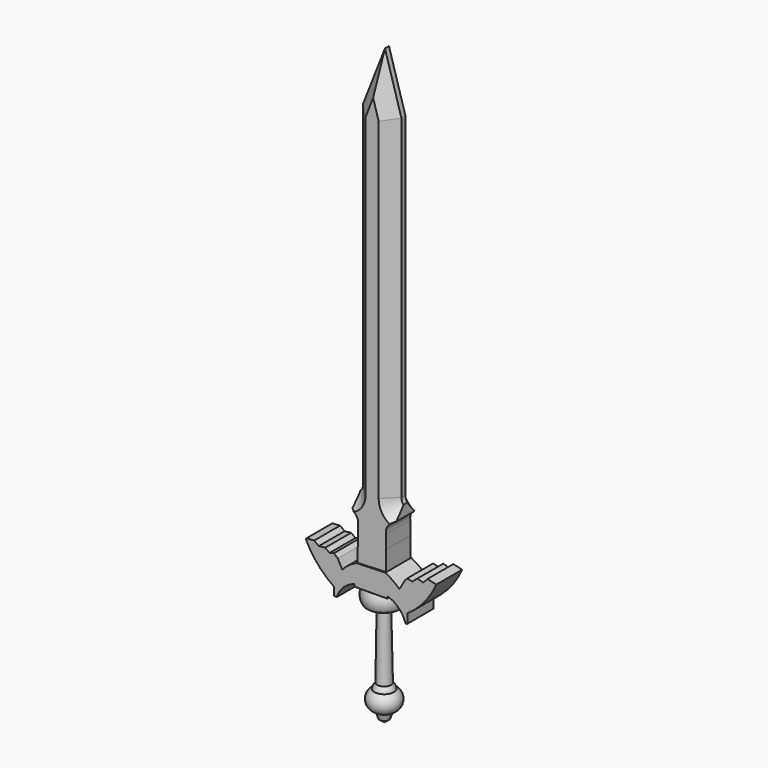
from build123d import *

# Parameters (mm, degrees)
F2_DEPTH     = 3.2512
F3_DEPTH     = 3.048
F4_T1_DEPTH  = 29.734621701
F4_T3_DEPTH  = 78.5599474126
F4_T5_DEPTH  = 29.3779460523
F4_T7_DEPTH  = 78.2899783824
F4_T10_ANGLE = 237.1999890444
F4_T12_ANGLE = 237.1999890444
F4_T14_ANGLE = 359.64
F4_T16_ANGLE = 359.64


# Not quite as in the source:
# - a fillet or chamfer that OpenCascade refuses, or shapes differently, is made with other operations: its cross-section is extruded or revolved along the edge and cut away or added


with BuildPart() as f1:
    # F0 (on Front) → F1 (revolve)
    with BuildSketch(Plane.XZ):
        with BuildLine():
            Line((-0.6275566491, -35.2181914225), (-3.9520729807, -35.2304723177))
            Line((-3.9520729807, -35.2304723177), (-4.0009869263, -35.190757364))
            ThreePointArc((-4.0009869263, -35.190757364), (-4.468403987, -36.7762535495), (-4.0009869263, -38.361749735))
            ThreePointArc((-4.0009869263, -38.361749735), (-2.9483659374, -38.9416202329), (-1.7635652912, -39.1428866466))
            Line((-1.7635652912, -39.1428866466), (-1.9475727458, -52.4323270698))
            Line((-1.9475727458, -52.4323270698), (-0.5639669494, -52.4323270698))
            Line((-0.5639669494, -52.4323270698), (-0.6275566491, -35.2181914225))
        make_face()
        with BuildLine():
            Line((-0.540195615, -58.8673782805), (-0.5639669494, -52.4323270698))
            Line((-0.5639669494, -52.4323270698), (-1.9475727458, -52.4323270698))
            ThreePointArc((-1.9475727458, -52.4323270698), (-2.3123844436, -52.9312298771), (-2.5166937266, -53.5145388027))
            ThreePointArc((-2.5166937266, -53.5145388027), (-3.6060607732, -55.2257600565), (-2.6693845284, -57.0251033684))
            ThreePointArc((-2.6693845284, -57.0251033684), (-2.3283302078, -57.2524646389), (-1.9475727458, -57.4042373379))
            Line((-1.9475727458, -57.4042373379), (-1.4987547765, -58.7614909788))
            Line((-1.4987547765, -58.7614909788), (-0.820128771, -59.2534937938))
            ThreePointArc((-0.820128771, -59.2534937938), (-0.6865028844, -59.3212967141), (-0.5384338847, -59.3442898632))
            Line((-0.5384338847, -59.3442898632), (-0.540195615, -58.8673782805))
        make_face()
    revolve(axis=Axis((-0.5851411479, 0, -46.7003370305), (0.0036940145, 0, -0.9999931771)))

    # F0 (on Front) → F2 (join, symmetric)
    with BuildSketch(Plane.XZ):
        with BuildLine():
            Line((2.2831694857, -30.7255659779), (-3.495863406, -30.9279132634))
            ThreePointArc((-3.495863406, -30.9279132634), (-5.0646851839, -31.7977900116), (-6.3840295188, -33.0131985247))
            Line((-6.3840295188, -33.0131985247), (-7.2957654484, -31.3216894865))
            Line((-7.2957654484, -31.3216894865), (-8.075539954, -30.6498836726))
            Line((-8.075539954, -30.6498836726), (-8.9392894879, -30.8778174222))
            Line((-8.9392894879, -30.8778174222), (-9.8150353879, -30.2420016378))
            Line((-9.8150353879, -30.2420016378), (-11.11066062, -30.3739625961))
            Line((-11.11066062, -30.3739625961), (-12.0343929157, -29.6901613474))
            Line((-12.0343929157, -29.6901613474), (-13.4499836713, -29.7861322761))
            ThreePointArc((-13.4499836713, -29.7861322761), (-13.6378178947, -29.8303732109), (-13.7259028852, -30.0020705909))
            ThreePointArc((-13.7259028852, -30.0020705909), (-11.3193803546, -33.6661550155), (-8.0515462905, -36.5881621838))
            Line((-8.0515462905, -36.5881621838), (-8.0515462905, -38.0517393351))
            ThreePointArc((-8.0515462905, -38.0517393351), (-7.9598069948, -38.2180289535), (-7.775626611, -38.1717048585))
            Line((-7.775626611, -38.1717048585), (-7.4828979958, -38.2224339632))
            ThreePointArc((-7.4828979958, -38.2224339632), (-6.1405359903, -36.0725037485), (-3.9553394628, -34.7883496227))
            Line((-3.9553394628, -34.7883496227), (-3.9520729807, -35.2304723177))
            Line((-3.9520729807, -35.2304723177), (-0.6275566491, -35.2181914225))
            Line((-0.6275566491, -35.2181914225), (2.6969596825, -35.2059105274))
            Line((2.6969596825, -35.2059105274), (2.6969596825, -34.7637757659))
            ThreePointArc((2.6969596825, -34.7637757659), (4.8915838758, -36.0317506602), (6.2497928845, -38.1717048585))
            ThreePointArc((6.2497928845, -38.1717048585), (6.5108954494, -38.4328074234), (6.7719980143, -38.1717048585))
            Line((6.7719980143, -38.1717048585), (6.7719980143, -36.4611186087))
            ThreePointArc((6.7719980143, -36.4611186087), (10.1347132538, -33.3799368553), (12.5336479489, -29.500936068))
            Line((12.5336479489, -29.500936068), (10.7419602573, -29.0980264544))
            Line((10.7419602573, -29.0980264544), (9.8929585313, -30.0165999209))
            Line((9.8929585313, -30.0165999209), (8.7400143966, -29.6748578548))
            Line((8.7400143966, -29.6748578548), (7.6542128809, -30.5570717901))
            Line((7.6542128809, -30.5570717901), (6.6702044569, -30.3195528686))
            Line((6.6702044569, -30.3195528686), (6.1612352729, -30.8963861316))
            Line((6.1612352729, -30.8963861316), (5.1093655638, -32.7286757529))
            ThreePointArc((5.1093655638, -32.7286757529), (3.7630618873, -31.6328804159), (2.2831694857, -30.7255659779))
        make_face()
    extrude(amount=F2_DEPTH, both=True)

    # F0 (on Front) → F3 (join, symmetric)
    with BuildSketch(Plane.XZ):
        with BuildLine():
            Line((-4.411068745, 48.9967949688), (-4.411068745, -18.4586253017))
            ThreePointArc((-4.411068745, -18.4586253017), (-4.5385726522, -19.078284844), (-4.9003679305, -19.5972640067))
            Line((-4.9003679305, -19.5972640067), (-4.9003679305, -21.9385232776))
            ThreePointArc((-4.9003679305, -21.9385232776), (-3.7434702801, -22.6334289507), (-3.4073905554, -23.9404700696))
            Line((-3.4073905554, -23.9404700696), (-3.4073905554, -26.6549736261))
            Line((-3.4073905554, -26.6549736261), (-3.495863406, -30.9279132634))
            Line((-3.495863406, -30.9279132634), (2.2831694857, -30.7255659779))
            Line((2.2831694857, -30.7255659779), (2.2591357119, -26.7228353769))
            Line((2.2591357119, -26.7228353769), (2.2591357119, -23.9404700696))
            ThreePointArc((2.2591357119, -23.9404700696), (2.5697152514, -22.5087595302), (3.7181819789, -21.5992107987))
            Line((3.7181819789, -21.5992107987), (3.7181819789, -19.3597450852))
            ThreePointArc((3.7181819789, -19.3597450852), (3.4148052065, -18.8087864436), (3.3097744472, -18.1886562715))
            Line((3.3097744472, -18.1886562715), (3.3097744472, 48.9967949688))
            Line((3.3097744472, 48.9967949688), (0, 60.2619871497))
            Line((0, 60.2619871497), (-4.411068745, 48.9967949688))
        make_face()
    extrude(amount=F3_DEPTH, both=True)

    # F4: chamfer of 2.54 on 8 edges, made by hand

    # F4_s2 → F4_t1 (cut)
    with BuildSketch(Plane(origin=(22.8412726569, 0, 58.3331027043), x_dir=(0, 1, 0), z_dir=(-0.3646108065, 0, -0.9311600076))):
        Polygon((3.048, -19.4321717346), (0.508, -21.9721717346), (3.048, -21.9721717346), align=None)
        Polygon((-3.048, -19.4321717346), (-0.508, -21.9721717346), (-3.048, -21.9721717346), align=None)
    extrude(amount=F4_T1_DEPTH, mode=Mode.SUBTRACT)

    # F4_s4 → F4_t3 (cut)
    with BuildSketch(Plane.XY.offset(-18.4586253017)):
        Polygon((-1.871068745, -3.048), (-4.411068745, -0.508), (-4.411068745, -3.048), align=None)
        Polygon((-1.871068745, 3.048), (-4.411068745, 0.508), (-4.411068745, 3.048), align=None)
    extrude(amount=F4_T3_DEPTH, mode=Mode.SUBTRACT)

    # F4_s6 → F4_t5 (cut)
    with BuildSketch(Plane(origin=(-9.8583580644, 0, 33.5540381846), x_dir=(0, 1, 0), z_dir=(-0.2818905922, 0, 0.9594465561))):
        Polygon((3.048, -14.4472872435), (0.508, -16.9872872435), (3.048, -16.9872872435), align=None)
        Polygon((-3.048, -14.4472872435), (-0.508, -16.9872872435), (-3.048, -16.9872872435), align=None)
    extrude(amount=F4_T5_DEPTH, mode=Mode.SUBTRACT)

    # F4_s8 → F4_t7 (cut)
    with BuildSketch(Plane.XY.offset(-18.1886562715)):
        Polygon((0.7697744472, 3.048), (3.3097744472, 0.508), (3.3097744472, 3.048), align=None)
        Polygon((0.7697744472, -3.048), (3.3097744472, -0.508), (3.3097744472, -3.048), align=None)
    extrude(amount=F4_T7_DEPTH, mode=Mode.SUBTRACT)

    # F4_s9 → F4_t10 (revolve, cut)
    with BuildSketch(Plane(origin=(11.9511811184, 0, -7.702013887), x_dir=(0, 1, 0), z_dir=(-0.8405664999, 0, 0.541708371))):
        Polygon((-3.048, 8.0524604286), (-0.508, 10.5924604286), (-3.048, 10.5924604286), align=None)
    revolve(axis=Axis((5.1929984357, -3.048, -18.1886562715), (0, 1, 0)), revolution_arc=F4_T10_ANGLE, mode=Mode.SUBTRACT)

    # F4_s11 → F4_t12 (revolve, cut)
    with BuildSketch(Plane(origin=(11.9511811184, 0, -7.702013887), x_dir=(0, 1, 0), z_dir=(-0.8405664999, 0, 0.541708371))):
        Polygon((3.048, 8.0524604286), (0.508, 10.5924604286), (3.048, 10.5924604286), align=None)
    revolve(axis=Axis((5.1929984357, 3.048, -18.1886562715), (0, 1, 0)), revolution_arc=F4_T12_ANGLE, mode=Mode.SUBTRACT)

    # F4_s13 → F4_t14 (revolve, cut)
    with BuildSketch(Plane.XY.offset(-18.4586253017)):
        Polygon((-1.871068745, 3.048), (-4.411068745, 0.508), (-4.411068745, 3.048), align=None)
    revolve(axis=Axis((-5.9805704311, 3.048, -18.4586253017), (0, 1, 0)), revolution_arc=F4_T14_ANGLE, mode=Mode.SUBTRACT)

    # F4_s15 → F4_t16 (revolve, cut)
    with BuildSketch(Plane.XY.offset(-18.4586253017)):
        Polygon((-1.871068745, -3.048), (-4.411068745, -0.508), (-4.411068745, -3.048), align=None)
    revolve(axis=Axis((-5.9805704311, -3.048, -18.4586253017), (0, 1, 0)), revolution_arc=F4_T16_ANGLE, mode=Mode.SUBTRACT)


solid = f1.part
